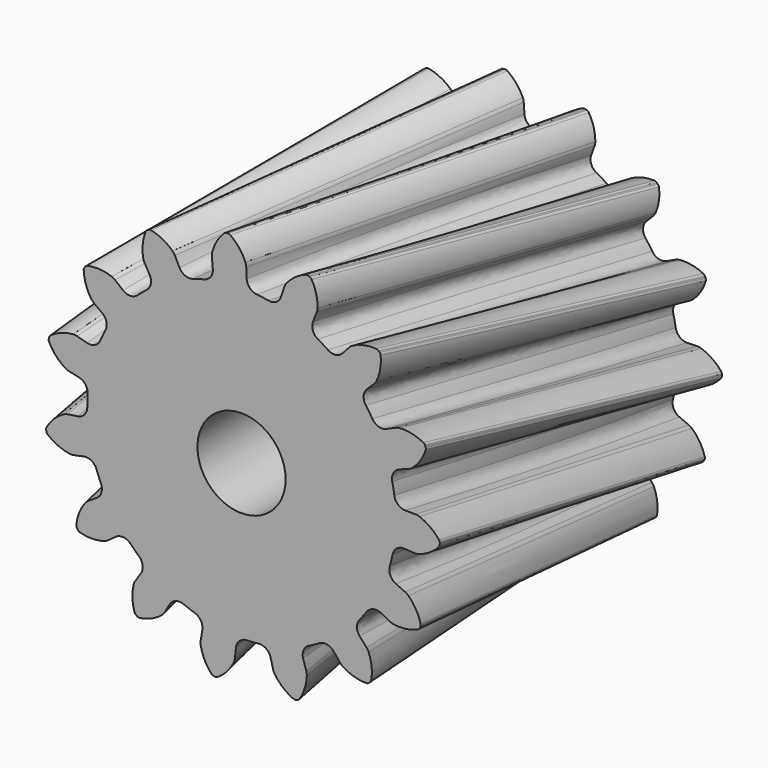
from build123d import *

# Parameters (mm, degrees)
F4_R      = 22.225
F5_DEPTH  = 50.8
F6_COUNT  = 15
F7_R      = 1.6002
F7_2_R    = 1.6002
F7_3_R    = 1.6002
F7_4_R    = 1.6002
F7_5_R    = 1.6002
F7_6_R    = 1.6002
F7_7_R    = 1.6002
F7_8_R    = 1.6002
F7_9_R    = 1.6002
F7_10_R   = 1.6002
F7_11_R   = 1.6002
F7_12_R   = 1.6002
F7_13_R   = 1.6002
F7_14_R   = 1.6002
F7_15_R   = 1.6002
F9_R      = 6.35
F10_DEPTH = 50.8010001


with BuildPart() as f3:
    # F2 (on offset) → F3 section 0
    with BuildSketch(Plane.XZ.offset(50.8)):
        with BuildLine():
            ThreePointArc((-12.5397047944, 18.3495620838), (-10.476792476, 19.6007001001), (-8.2904165571, 20.6208539665))
            Line((-8.2904165571, 20.6208539665), (-9.6057788379, 23.2388833737))
            ThreePointArc((-9.6057788379, 23.2388833737), (-9.7482442688, 23.4708599132), (-9.9279695822, 23.675330756))
            ThreePointArc((-9.9279695822, 23.675330756), (-11.3594007898, 24.7083191202), (-13.0198956146, 25.3073326422))
            ThreePointArc((-13.0198956146, 25.3073326422), (-13.193433189, 25.3134115305), (-13.3588799898, 25.2606896309))
            Line((-13.3588799898, 25.2606896309), (-13.4709229572, 25.2023242382))
            Line((-13.4709229572, 25.2023242382), (-13.5816997451, 25.1415899904))
            ThreePointArc((-13.5816997451, 25.1415899904), (-13.7174537202, 25.0333167211), (-13.8088116199, 24.885648252))
            ThreePointArc((-13.8088116199, 24.885648252), (-14.2332715757, 23.1722031818), (-14.1696337106, 21.4081140444))
            ThreePointArc((-14.1696337106, 21.4081140444), (-14.0994724525, 21.1450799939), (-13.9857405618, 20.8977450573))
            Line((-13.9857405618, 20.8977450573), (-12.5397047944, 18.3495620838))
        make_face()
    # F0 (on Front) → F3 section 1
    with BuildSketch(Plane.XZ):
        with BuildLine():
            ThreePointArc((-4.5631032027, 21.7515221114), (-2.1784309438, 22.1179805503), (0.2319130011, 22.2237899864))
            Line((0.2319130011, 22.2237899864), (0.0185531916, 25.1459011236))
            ThreePointArc((0.0185531916, 25.1459011236), (-0.0242941257, 25.4147386606), (-0.1120910603, 25.6724229871))
            ThreePointArc((-0.1120910603, 25.6724229871), (-1.0392535225, 27.1745648018), (-2.3441181542, 28.3634249934))
            ThreePointArc((-2.3441181542, 28.3634249934), (-2.5021196775, 28.4354511085), (-2.675148388, 28.4500561742))
            Line((-2.675148388, 28.4500561742), (-2.8009980611, 28.4390105698))
            Line((-2.8009980611, 28.4390105698), (-2.9265844586, 28.4252918828))
            ThreePointArc((-2.9265844586, 28.4252918828), (-3.0934391639, 28.3772112224), (-3.2343531342, 28.2757445009))
            ThreePointArc((-3.2343531342, 28.2757445009), (-4.2822100404, 26.8551614633), (-4.8985040054, 25.2010024591))
            ThreePointArc((-4.8985040054, 25.2010024591), (-4.9343422284, 24.9311411324), (-4.9239186448, 24.6591101364))
            Line((-4.9239186448, 24.6591101364), (-4.5631032027, 21.7515221114))
        make_face()
    loft()

    # F4 (on Front) → F5 (join, through all)
    with BuildSketch(Plane.XZ):
        Circle(F4_R)
    extrude(amount=F5_DEPTH)


with BuildPart() as f6_1:
    # F6: instance of F3
    add(f3.part.rotate(Axis((0, 0, 0), (0, 1, 0)), 1 * 360 / F6_COUNT))

    # F7#2
    f7_2_edges = [f6_1.edges().sort_by_distance(p)[0] for p in [
        (0.384546, -25.405912, 22.221673),
        (5.096731, -25.396996, 21.632706),
    ]]
    fillet(f7_2_edges, radius=F7_2_R)


with BuildPart() as f6_2:
    # F6: instance of F3
    add(f3.part.rotate(Axis((0, 0, 0), (0, 1, 0)), 2 * 360 / F6_COUNT))

    # F7#3
    f7_3_edges = [f6_2.edges().sort_by_distance(p)[0] for p in [
        (9.389669, -25.405912, 20.144099),
        (13.45491, -25.396996, 17.689433),
    ]]
    fillet(f7_3_edges, radius=F7_3_R)


with BuildPart() as f6_3:
    # F6: instance of F3
    add(f3.part.rotate(Axis((0, 0, 0), (0, 1, 0)), 3 * 360 / F6_COUNT))

    # F7#4
    f7_4_edges = [f6_3.edges().sort_by_distance(p)[0] for p in [
        (16.771233, -25.405912, 14.583428),
        (19.486612, -25.396996, 10.687496),
    ]]
    fillet(f7_4_edges, radius=F7_4_R)


with BuildPart() as f6_4:
    # F6: instance of F3
    add(f3.part.rotate(Axis((0, 0, 0), (0, 1, 0)), 4 * 360 / F6_COUNT))

    # F7#5
    f7_5_edges = [f6_4.edges().sort_by_distance(p)[0] for p in [
        (21.252898, -25.405912, 6.50115),
        (22.148902, -25.396996, 1.837594),
    ]]
    fillet(f7_5_edges, radius=F7_5_R)


with BuildPart() as f6_5:
    # F6: instance of F3
    add(f3.part.rotate(Axis((0, 0, 0), (0, 1, 0)), 5 * 360 / F6_COUNT))

    # F7#6
    f7_6_edges = [f6_5.edges().sort_by_distance(p)[0] for p in [
        (22.059744, -25.405912, -2.705237),
        (20.981446, -25.396996, -7.330044),
    ]]
    fillet(f7_6_edges, radius=F7_6_R)


with BuildPart() as f6_6:
    # F6: instance of F3
    add(f3.part.rotate(Axis((0, 0, 0), (0, 1, 0)), 6 * 360 / F6_COUNT))

    # F7#7
    f7_7_edges = [f6_6.edges().sort_by_distance(p)[0] for p in [
        (19.05226, -25.405912, -11.443863),
        (16.186107, -25.396996, -15.230252),
    ]]
    fillet(f7_7_edges, radius=F7_7_R)


with BuildPart() as f6_7:
    # F6: instance of F3
    add(f3.part.rotate(Axis((0, 0, 0), (0, 1, 0)), 7 * 360 / F6_COUNT))

    # F7#8
    f7_8_edges = [f6_7.edges().sort_by_distance(p)[0] for p in [
        (12.750467, -25.405912, -18.203742),
        (8.592043, -25.396996, -20.49701),
    ]]
    fillet(f7_8_edges, radius=F7_8_R)


with BuildPart() as f6_8:
    # F6: instance of F3
    add(f3.part.rotate(Axis((0, 0, 0), (0, 1, 0)), 8 * 360 / F6_COUNT))

    # F7#9
    f7_9_edges = [f6_8.edges().sort_by_distance(p)[0] for p in [
        (4.244003, -25.405912, -21.816028),
        (-0.487663, -25.396996, -22.219649),
    ]]
    fillet(f7_9_edges, radius=F7_9_R)


with BuildPart() as f6_9:
    # F6: instance of F3
    add(f3.part.rotate(Axis((0, 0, 0), (0, 1, 0)), 9 * 360 / F6_COUNT))

    # F7#10
    f7_10_edges = [f6_9.edges().sort_by_distance(p)[0] for p in [
        (-4.996288, -25.405912, -21.656124),
        (-9.483048, -25.396996, -20.100309),
    ]]
    fillet(f7_10_edges, radius=F7_10_R)


with BuildPart() as f6_10:
    # F6: instance of F3
    add(f3.part.rotate(Axis((0, 0, 0), (0, 1, 0)), 10 * 360 / F6_COUNT))

    # F7#11
    f7_11_edges = [f6_10.edges().sort_by_distance(p)[0] for p in [
        (-13.372676, -25.405912, -17.751681),
        (-16.838728, -25.396996, -14.505443),
    ]]
    fillet(f7_11_edges, radius=F7_11_R)


with BuildPart() as f6_11:
    # F6: instance of F3
    add(f3.part.rotate(Axis((0, 0, 0), (0, 1, 0)), 11 * 360 / F6_COUNT))

    # F7#12
    f7_12_edges = [f6_11.edges().sort_by_distance(p)[0] for p in [
        (-19.436806, -25.405912, -10.77781),
        (-21.282838, -25.396996, -6.402454),
    ]]
    fillet(f7_12_edges, radius=F7_12_R)


with BuildPart() as f6_12:
    # F6: instance of F3
    add(f3.part.rotate(Axis((0, 0, 0), (0, 1, 0)), 12 * 360 / F6_COUNT))

    # F7#13
    f7_13_edges = [f6_12.edges().sort_by_distance(p)[0] for p in [
        (-22.140136, -25.405912, -1.940358),
        (-22.046953, -25.396996, 2.807578),
    ]]
    fillet(f7_13_edges, radius=F7_13_R)


with BuildPart() as f6_13:
    # F6: instance of F3
    add(f3.part.rotate(Axis((0, 0, 0), (0, 1, 0)), 13 * 360 / F6_COUNT))

    # F7#14
    f7_14_edges = [f6_13.edges().sort_by_distance(p)[0] for p in [
        (-21.015236, -25.405912, 7.2326),
        (-18.998949, -25.396996, 11.532153),
    ]]
    fillet(f7_14_edges, radius=F7_14_R)


with BuildPart() as f6_14:
    # F6: instance of F3
    add(f3.part.rotate(Axis((0, 0, 0), (0, 1, 0)), 14 * 360 / F6_COUNT))

    # F7#15
    f7_15_edges = [f6_14.edges().sort_by_distance(p)[0] for p in [
        (-16.25661, -25.405912, 15.154975),
        (-12.665854, -25.396996, 18.262715),
    ]]
    fillet(f7_15_edges, radius=F7_15_R)


with BuildPart() as f3_1:
    add(f3.part)

    # F7
    f7_edges = [f3_1.edges().sort_by_distance(p)[0] for p in [
        (-8.687068, -25.405912, 20.456917),
        (-4.142718, -25.396996, 21.835487),
    ]]
    fillet(f7_edges, radius=F7_R)


with BuildPart() as f6_14_1:
    add(f6_14.part)

    # F8: union F3, F6_1, F6_2, F6_3, F6_4, F6_5, F6_6, F6_7, F6_9, F6_10, F6_11, F6_12, F6_13, F6_8
    add(f3_1.part)
    add(f6_1.part)
    add(f6_2.part)
    add(f6_3.part)
    add(f6_4.part)
    add(f6_5.part)
    add(f6_6.part)
    add(f6_7.part)
    add(f6_9.part)
    add(f6_10.part)
    add(f6_11.part)
    add(f6_12.part)
    add(f6_13.part)
    add(f6_8.part)

    # F9 (on face) → F10 (cut, through all)
    with BuildSketch(Plane.XZ.offset(50.8)):
        Circle(F9_R)
    extrude(amount=-F10_DEPTH, mode=Mode.SUBTRACT)


solid = f6_14_1.part
